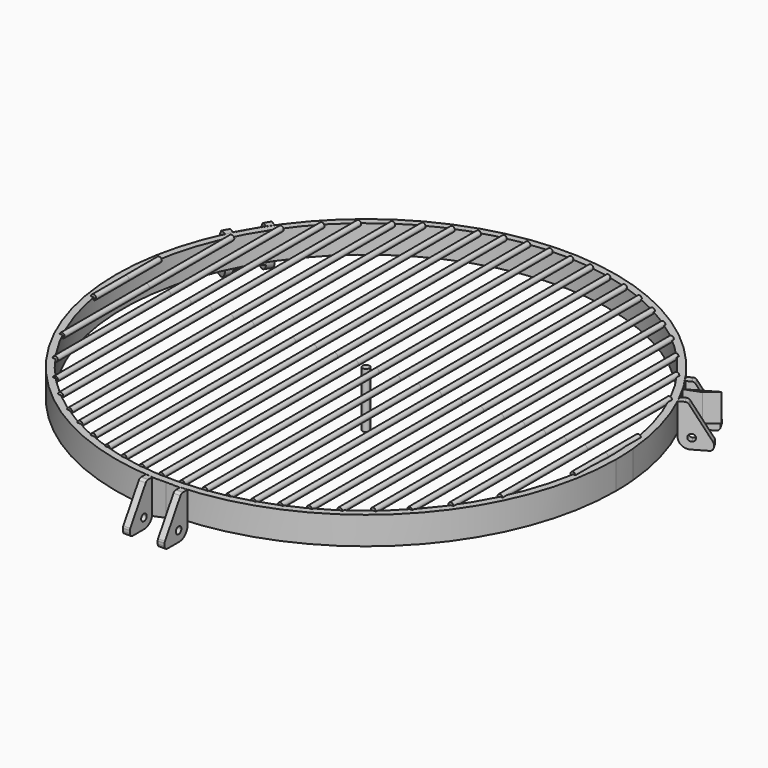
from build123d import *

# Parameters (mm, degrees)
F1_DEPTH  = 25.4
F3_R      = 2.38125
F4_DEPTH  = 222.0468
F5_DEPTH  = 222.0468
F6_DEPTH  = 222.0468
F7_DEPTH  = 222.0468
F8_DEPTH  = 220.40596
F9_DEPTH  = 220.40596
F10_DEPTH = 220.40596
F11_DEPTH = 220.40596
F12_DEPTH = 217.08618
F13_DEPTH = 217.08618
F14_DEPTH = 217.08618
F15_DEPTH = 217.08618
F16_DEPTH = 212.0138
F17_DEPTH = 212.0138
F18_DEPTH = 212.0138
F19_DEPTH = 212.0138
F20_DEPTH = 205.05166
F21_DEPTH = 205.05166
F22_DEPTH = 205.05166
F23_DEPTH = 205.05166
F24_DEPTH = 195.9864
F25_DEPTH = 196.00418
F26_DEPTH = 196.00418
F27_DEPTH = 196.00418
F28_DEPTH = 184.55894
F29_DEPTH = 184.55894
F30_DEPTH = 184.55894
F31_DEPTH = 184.55894
F32_DEPTH = 170.24096
F33_DEPTH = 170.24096
F34_DEPTH = 170.24096
F35_DEPTH = 170.24096
F36_DEPTH = 152.2349
F37_DEPTH = 152.2349
F38_DEPTH = 152.2349
F39_DEPTH = 152.2349
F40_DEPTH = 129.00914
F41_DEPTH = 129.00914
F42_DEPTH = 129.00914
F43_DEPTH = 129.00914
F44_DEPTH = 96.8756
F45_DEPTH = 96.8756
F46_DEPTH = 96.8756
F47_DEPTH = 96.8756
F48_DEPTH = 37.43198
F49_DEPTH = 37.43198
F50_DEPTH = 37.43198
F51_DEPTH = 37.43198
F53_DEPTH = 38.1
F54_DEPTH = 25.4
F56_R     = 9.525
F57_DEPTH = 6.35
F58_R     = 3.175
F60_DEPTH = 50.8
F61_ANGLE = 120
F62_ANGLE = -120


with BuildPart() as f1:
    # F0 (on Top) → F1 (new body)
    with BuildSketch(Plane.XY):
        with BuildLine():
            ThreePointArc((-131.2249606136, 187.1843201552), (-227.7188567513, -20.0519894244), (-96.4938961377, -207.2363095796))
            Line((-96.4938961377, -207.2363095796), (-93.8135101339, -201.4797454246))
            ThreePointArc((-93.8135101339, -201.4797454246), (-221.3933329527, -19.4949897181), (-127.5798228187, 181.9847557065))
            Line((-127.5798228187, 181.9847557065), (-131.2249606136, 187.1843201552))
        make_face()
        with BuildLine():
            ThreePointArc((-96.4938961377, -207.2363095796), (122.8809491803, -192.7647071654), (228.6, 0))
            ThreePointArc((228.6, 0), (228.3796079484, 10.0356700486), (227.7188567513, 20.0519894244))
            Line((227.7188567513, 20.0519894244), (221.3933329527, 19.4949897181))
            ThreePointArc((221.3933329527, 19.4949897181), (222.0357299499, 9.7569014362), (222.25, 0))
            ThreePointArc((222.25, 0), (119.4675894809, -187.4101319663), (-93.8135101339, -201.4797454246))
            Line((-93.8135101339, -201.4797454246), (-96.4938961377, -207.2363095796))
        make_face()
        with BuildLine():
            Line((221.3933329527, 19.4949897181), (227.7188567513, 20.0519894244))
            ThreePointArc((227.7188567513, 20.0519894244), (96.4938961377, 207.2363095796), (-131.2249606136, 187.1843201552))
            Line((-131.2249606136, 187.1843201552), (-127.5798228187, 181.9847557065))
            ThreePointArc((-127.5798228187, 181.9847557065), (93.8135101339, 201.4797454246), (221.3933329527, 19.4949897181))
        make_face()
    extrude(amount=-F1_DEPTH)


with BuildPart() as f4:
    # F3 (on Front) → F4 (new body)
    with BuildSketch(Plane.XZ):
        with Locations((9.5708072186, -0.3158553445)):
            Circle(F3_R)
    extrude(amount=-F4_DEPTH)

    # F3 (on Front) → F5 (join)
    with BuildSketch(Plane.XZ):
        with Locations((9.5708072186, -0.3158553445)):
            Circle(F3_R)
    extrude(amount=F5_DEPTH)


with BuildPart() as f6:
    # F3 (on Front) → F6 (new body)
    with BuildSketch(Plane.XZ):
        with Locations((-9.425139986, -0.106897467)):
            Circle(F3_R)
    extrude(amount=F6_DEPTH)


with BuildPart() as f7:
    # F3 (on Front) → F7 (new body)
    with BuildSketch(Plane.XZ):
        with Locations((-9.425139986, -0.106897467)):
            Circle(F3_R)
    extrude(amount=-F7_DEPTH)


with BuildPart() as f8:
    # F3 (on Front) → F8 (new body)
    with BuildSketch(Plane.XZ):
        with Locations((-28.4335520118, -0.180243529)):
            Circle(F3_R)
    extrude(amount=F8_DEPTH)


with BuildPart() as f9:
    # F3 (on Front) → F9 (new body)
    with BuildSketch(Plane.XZ):
        with Locations((29.0328394622, 0.0237040113)):
            Circle(F3_R)
    extrude(amount=F9_DEPTH)


with BuildPart() as f10:
    # F3 (on Front) → F10 (new body)
    with BuildSketch(Plane.XZ):
        with Locations((29.0328394622, 0.0237040113)):
            Circle(F3_R)
    extrude(amount=-F10_DEPTH)


with BuildPart() as f11:
    # F3 (on Front) → F11 (new body)
    with BuildSketch(Plane.XZ):
        with Locations((-28.4335520118, -0.180243529)):
            Circle(F3_R)
    extrude(amount=-F11_DEPTH)


with BuildPart() as f12:
    # F3 (on Front) → F12 (new body)
    with BuildSketch(Plane.XZ):
        with Locations((47.5846938789, -0.6066233036)):
            Circle(F3_R)
    extrude(amount=F12_DEPTH)


with BuildPart() as f13:
    # F3 (on Front) → F13 (new body)
    with BuildSketch(Plane.XZ):
        with Locations((47.5846938789, -0.6066233036)):
            Circle(F3_R)
    extrude(amount=-F13_DEPTH)


with BuildPart() as f14:
    # F3 (on Front) → F14 (new body)
    with BuildSketch(Plane.XZ):
        with Locations((-47.4231056869, 0.0243091217)):
            Circle(F3_R)
    extrude(amount=F14_DEPTH)


with BuildPart() as f15:
    # F3 (on Front) → F15 (new body)
    with BuildSketch(Plane.XZ):
        with Locations((-47.4231056869, 0.0243091217)):
            Circle(F3_R)
    extrude(amount=-F15_DEPTH)


with BuildPart() as f16:
    # F3 (on Front) → F16 (new body)
    with BuildSketch(Plane.XZ):
        with Locations((66.6127800941, -0.4029138654)):
            Circle(F3_R)
    extrude(amount=F16_DEPTH)


with BuildPart() as f17:
    # F3 (on Front) → F17 (new body)
    with BuildSketch(Plane.XZ):
        with Locations((-66.8880864978, -0.4602428235)):
            Circle(F3_R)
    extrude(amount=F17_DEPTH)


with BuildPart() as f18:
    # F3 (on Front) → F18 (new body)
    with BuildSketch(Plane.XZ):
        with Locations((66.6127800941, -0.4029138654)):
            Circle(F3_R)
    extrude(amount=-F18_DEPTH)


with BuildPart() as f19:
    # F3 (on Front) → F19 (new body)
    with BuildSketch(Plane.XZ):
        with Locations((-66.8880864978, -0.4602428235)):
            Circle(F3_R)
    extrude(amount=-F19_DEPTH)


with BuildPart() as f20:
    # F3 (on Front) → F20 (new body)
    with BuildSketch(Plane.XZ):
        with Locations((85.7855156064, -0.15390724)):
            Circle(F3_R)
    extrude(amount=F20_DEPTH)


with BuildPart() as f21:
    # F3 (on Front) → F21 (new body)
    with BuildSketch(Plane.XZ):
        with Locations((-85.2940529585, -0.0779687107)):
            Circle(F3_R)
    extrude(amount=F21_DEPTH)


with BuildPart() as f22:
    # F3 (on Front) → F22 (new body)
    with BuildSketch(Plane.XZ):
        with Locations((85.7855156064, -0.15390724)):
            Circle(F3_R)
    extrude(amount=-F22_DEPTH)


with BuildPart() as f23:
    # F3 (on Front) → F23 (new body)
    with BuildSketch(Plane.XZ):
        with Locations((-85.2940529585, -0.0779687107)):
            Circle(F3_R)
    extrude(amount=-F23_DEPTH)


with BuildPart() as f24:
    # F3 (on Front) → F24 (new body)
    with BuildSketch(Plane.XZ):
        with Locations((104.9413457513, -0.1841801713)):
            Circle(F3_R)
    extrude(amount=F24_DEPTH)


with BuildPart() as f25:
    # F3 (on Front) → F25 (new body)
    with BuildSketch(Plane.XZ):
        with Locations((104.9413457513, -0.1841801713)):
            Circle(F3_R)
    extrude(amount=-F25_DEPTH)


with BuildPart() as f26:
    # F3 (on Front) → F26 (new body)
    with BuildSketch(Plane.XZ):
        with Locations((-104.7213003039, -0.0067136111)):
            Circle(F3_R)
    extrude(amount=F26_DEPTH)


with BuildPart() as f27:
    # F3 (on Front) → F27 (new body)
    with BuildSketch(Plane.XZ):
        with Locations((-104.7213003039, -0.0067136111)):
            Circle(F3_R)
    extrude(amount=-F27_DEPTH)


with BuildPart() as f28:
    # F3 (on Front) → F28 (new body)
    with BuildSketch(Plane.XZ):
        with Locations((-123.4662309289, -0.4080603539)):
            Circle(F3_R)
    extrude(amount=F28_DEPTH)


with BuildPart() as f29:
    # F3 (on Front) → F29 (new body)
    with BuildSketch(Plane.XZ):
        with Locations((-123.4662309289, -0.4080603539)):
            Circle(F3_R)
    extrude(amount=-F29_DEPTH)


with BuildPart() as f30:
    # F3 (on Front) → F30 (new body)
    with BuildSketch(Plane.XZ):
        with Locations((123.67169559, -0.2106657048)):
            Circle(F3_R)
    extrude(amount=-F30_DEPTH)


with BuildPart() as f31:
    # F3 (on Front) → F31 (new body)
    with BuildSketch(Plane.XZ):
        with Locations((123.67169559, -0.2106657048)):
            Circle(F3_R)
    extrude(amount=F31_DEPTH)


with BuildPart() as f32:
    # F3 (on Front) → F32 (new body)
    with BuildSketch(Plane.XZ):
        with Locations((-143.0111080408, 0.0356082346)):
            Circle(F3_R)
    extrude(amount=-F32_DEPTH)


with BuildPart() as f33:
    # F3 (on Front) → F33 (new body)
    with BuildSketch(Plane.XZ):
        with Locations((-143.0111080408, 0.0356082346)):
            Circle(F3_R)
    extrude(amount=F33_DEPTH)


with BuildPart() as f34:
    # F3 (on Front) → F34 (new body)
    with BuildSketch(Plane.XZ):
        with Locations((142.8444236517, 0.0383409097)):
            Circle(F3_R)
    extrude(amount=-F34_DEPTH)


with BuildPart() as f35:
    # F3 (on Front) → F35 (new body)
    with BuildSketch(Plane.XZ):
        with Locations((142.8444236517, 0.0383409097)):
            Circle(F3_R)
    extrude(amount=F35_DEPTH)


with BuildPart() as f36:
    # F3 (on Front) → F36 (new body)
    with BuildSketch(Plane.XZ):
        with Locations((-162.2031480074, -0.6379687111)):
            Circle(F3_R)
    extrude(amount=F36_DEPTH)


with BuildPart() as f37:
    # F3 (on Front) → F37 (new body)
    with BuildSketch(Plane.XZ):
        with Locations((161.7707908154, -0.528559438)):
            Circle(F3_R)
    extrude(amount=-F37_DEPTH)


with BuildPart() as f38:
    # F3 (on Front) → F38 (new body)
    with BuildSketch(Plane.XZ):
        with Locations((161.7707908154, -0.528559438)):
            Circle(F3_R)
    extrude(amount=F38_DEPTH)


with BuildPart() as f39:
    # F3 (on Front) → F39 (new body)
    with BuildSketch(Plane.XZ):
        with Locations((-162.2031480074, -0.6379687111)):
            Circle(F3_R)
    extrude(amount=-F39_DEPTH)


with BuildPart() as f40:
    # F3 (on Front) → F40 (new body)
    with BuildSketch(Plane.XZ):
        with Locations((-180.8726340532, 0.0722792684)):
            Circle(F3_R)
    extrude(amount=F40_DEPTH)


with BuildPart() as f41:
    # F3 (on Front) → F41 (new body)
    with BuildSketch(Plane.XZ):
        with Locations((-180.8726340532, 0.0722792684)):
            Circle(F3_R)
    extrude(amount=-F41_DEPTH)


with BuildPart() as f42:
    # F3 (on Front) → F42 (new body)
    with BuildSketch(Plane.XZ):
        with Locations((180.8151602745, -0.1261264406)):
            Circle(F3_R)
    extrude(amount=F42_DEPTH)


with BuildPart() as f43:
    # F3 (on Front) → F43 (new body)
    with BuildSketch(Plane.XZ):
        with Locations((180.8151602745, -0.1261264406)):
            Circle(F3_R)
    extrude(amount=-F43_DEPTH)


with BuildPart() as f44:
    # F3 (on Front) → F44 (new body)
    with BuildSketch(Plane.XZ):
        with Locations((-200.3470212221, -0.5512023927)):
            Circle(F3_R)
    extrude(amount=F44_DEPTH)


with BuildPart() as f45:
    # F3 (on Front) → F45 (new body)
    with BuildSketch(Plane.XZ):
        with Locations((-200.3470212221, -0.5512023927)):
            Circle(F3_R)
    extrude(amount=-F45_DEPTH)


with BuildPart() as f46:
    # F3 (on Front) → F46 (new body)
    with BuildSketch(Plane.XZ):
        with Locations((199.9530941248, -0.3436789557)):
            Circle(F3_R)
    extrude(amount=F46_DEPTH)


with BuildPart() as f47:
    # F3 (on Front) → F47 (new body)
    with BuildSketch(Plane.XZ):
        with Locations((199.9530941248, -0.3436789557)):
            Circle(F3_R)
    extrude(amount=-F47_DEPTH)


with BuildPart() as f48:
    # F3 (on Front) → F48 (new body)
    with BuildSketch(Plane.XZ):
        with Locations((-219.075, 0)):
            Circle(F3_R)
    extrude(amount=F48_DEPTH)


with BuildPart() as f49:
    # F3 (on Front) → F49 (new body)
    with BuildSketch(Plane.XZ):
        with Locations((-219.075, 0)):
            Circle(F3_R)
    extrude(amount=-F49_DEPTH)


with BuildPart() as f50:
    # F3 (on Front) → F50 (new body)
    with BuildSketch(Plane.XZ):
        with Locations((218.9682126045, -0.3423732996)):
            Circle(F3_R)
    extrude(amount=F50_DEPTH)


with BuildPart() as f51:
    # F3 (on Front) → F51 (new body)
    with BuildSketch(Plane.XZ):
        with Locations((218.9682126045, -0.3423732996)):
            Circle(F3_R)
    extrude(amount=-F51_DEPTH)


with BuildPart() as f53:
    # F52 (on face) → F53 (new body)
    with BuildSketch(Plane.XY):
        with BuildLine():
            ThreePointArc((187.7598020629, 130.4002175201), (193.0345343543, 122.456639455), (197.9734073051, 114.3))
            Line((197.9734073051, 114.3), (191.6234073051, 125.2985226281))
            Line((191.6234073051, 125.2985226281), (213.6204525612, 137.9985226281))
            Line((213.6204525612, 137.9985226281), (210.4454525612, 143.4977839421))
            Line((210.4454525612, 143.4977839421), (187.7598020629, 130.4002175201))
        make_face()
    extrude(amount=-F53_DEPTH)

    # F56
    f56_edges = [f53.edges().sort_by_distance(p)[0] for p in [
        (193.034534, 122.456639, -38.1),
    ]]
    fillet(f56_edges, radius=F56_R)

    # F55 (on face) → F57 (cut)
    with BuildSketch(Plane(origin=(-9.525, 16.4977839421, 0), x_dir=(-0.8660254038, -0.5, 0), z_dir=(-0.5, 0.8660254038, 0))):
        Polygon((-234.95, 0), (-254, 0), (-254, -31.75), align=None)
        with BuildLine():
            ThreePointArc((-237.9648671561, -31.75), (-235.7198031258, -30.8200640303), (-234.7898671561, -28.575))
            Line((-234.7898671561, -28.575), (-237.9648671561, -28.575))
            Line((-237.9648671561, -28.575), (-237.9648671561, -31.75))
        make_face()
        with BuildLine():
            Line((-237.9648671561, -28.575), (-234.7898671561, -28.575))
            ThreePointArc((-234.7898671561, -28.575), (-240.2099311863, -26.3299359697), (-237.9648671561, -31.75))
            Line((-237.9648671561, -31.75), (-237.9648671561, -28.575))
        make_face()
    extrude(amount=-F57_DEPTH, mode=Mode.SUBTRACT)

    # F58
    f58_edges = [f53.edges().sort_by_distance(p)[0] for p in [
        (195.535169, 131.223153, 0),
        (212.032953, 140.748153, -31.75),
        (212.032953, 140.748153, -38.1),
    ]]
    fillet(f58_edges, radius=F58_R)


with BuildPart() as f54:
    # F52 (on face) → F54 (new body)
    with BuildSketch(Plane.XY):
        Polygon((222.2692602019, 128.3272172101), (197.9734073051, 114.3), (212.0490968227, 119.5174306631), align=None)
    extrude(amount=-F54_DEPTH)


with BuildPart() as f59_1:
    # F59: instance of F53
    add(f53.part.mirror(Plane(origin=(210.1213337535, 121.3136086051, -12.7), x_dir=(-0.8660254038, -0.5, 0), z_dir=(-0.5, 0.8660254038, 0))))


with BuildPart() as f60:
    # F0 (on Top) → F60 (new body)
    with BuildSketch(Plane.XY):
        with BuildLine():
            ThreePointArc((3.175, 0), (3.1719389993, 0.1393843062), (3.1627618993, 0.2784998531))
            Line((3.1627618993, 0.2784998531), (0, 0))
            Line((0, 0), (-1.3401930019, -2.8782820775))
            ThreePointArc((-1.3401930019, -2.8782820775), (1.7066798497, -2.6772875995), (3.175, 0))
        make_face()
        with BuildLine():
            ThreePointArc((-1.8225688974, 2.5997822244), (-3.1627618993, -0.2784998531), (-1.3401930019, -2.8782820775))
            Line((-1.3401930019, -2.8782820775), (0, 0))
            Line((0, 0), (-1.8225688974, 2.5997822244))
        make_face()
        with BuildLine():
            Line((0, 0), (3.1627618993, 0.2784998531))
            ThreePointArc((3.1627618993, 0.2784998531), (1.3401930019, 2.8782820775), (-1.8225688974, 2.5997822244))
            Line((-1.8225688974, 2.5997822244), (0, 0))
        make_face()
    extrude(amount=-F60_DEPTH)


with BuildPart() as f61_1:
    # F61: copy of F53
    add(f53.part.rotate(Axis((0, 0, 0), (0, 0, 1)), F61_ANGLE))


with BuildPart() as f61_2:
    # F61: copy of F59_1
    add(f59_1.part.rotate(Axis((0, 0, 0), (0, 0, 1)), F61_ANGLE))


with BuildPart() as f62_1:
    # F62: copy of F53
    add(f53.part.rotate(Axis((0, 0, 0), (0, 0, 1)), F62_ANGLE))


with BuildPart() as f62_2:
    # F62: copy of F59_1
    add(f59_1.part.rotate(Axis((0, 0, 0), (0, 0, 1)), F62_ANGLE))


solid = Compound([f1.part, f4.part, f6.part, f7.part, f8.part, f9.part, f10.part, f11.part, f12.part, f13.part, f14.part, f15.part, f16.part, f17.part, f18.part, f19.part, f20.part, f21.part, f22.part, f23.part, f24.part, f25.part, f26.part, f27.part, f28.part, f29.part, f30.part, f31.part, f32.part, f33.part, f34.part, f35.part, f36.part, f37.part, f38.part, f39.part, f40.part, f41.part, f42.part, f43.part, f44.part, f45.part, f46.part, f47.part, f48.part, f49.part, f50.part, f51.part, f53.part, f54.part, f59_1.part, f60.part, f61_1.part, f61_2.part, f62_1.part, f62_2.part])
